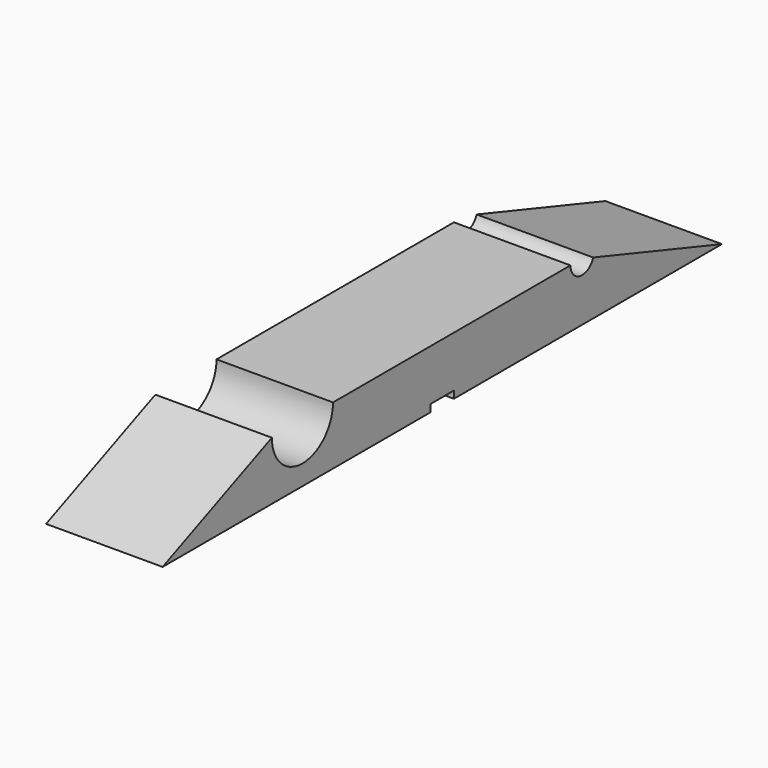
from build123d import *

# Parameters (mm, degrees)
F1_DEPTH = 25.4


# Not quite as in the source:
# - a feature names something its author has since deleted; it is built from what else it names


with BuildPart() as f1:
    # F0 (on Right) → F1 (new body)
    with BuildSketch(Plane.YZ):
        with BuildLine():
            ThreePointArc((41.1120694713, 5.3459768429), (37.5914213785, 3.215997322), (34.925, 6.35))
            Line((34.925, 6.35), (3.175, 6.35))
            Line((3.175, 6.35), (-3.175, 6.35))
            Line((-3.175, 6.35), (-29.7688, 6.35))
            ThreePointArc((-29.7688, 6.35), (-38.1, -1.9812), (-46.4312, 6.35))
            Line((-46.4312, 6.35), (-76.2, -6.35))
            Line((-76.2, -6.35), (-3.175, -6.35))
            Line((-3.175, -6.35), (-3.175, -4.7625))
            Line((-3.175, -4.7625), (0, -4.7625))
            Line((0, -4.7625), (3.175, -4.7625))
            Line((3.175, -4.7625), (3.175, -6.35))
            Line((3.175, -6.35), (76.2, -6.35))
            Line((76.2, -6.35), (41.1120694713, 5.3459768429))
        make_face()
    extrude(amount=F1_DEPTH)


solid = f1.part
